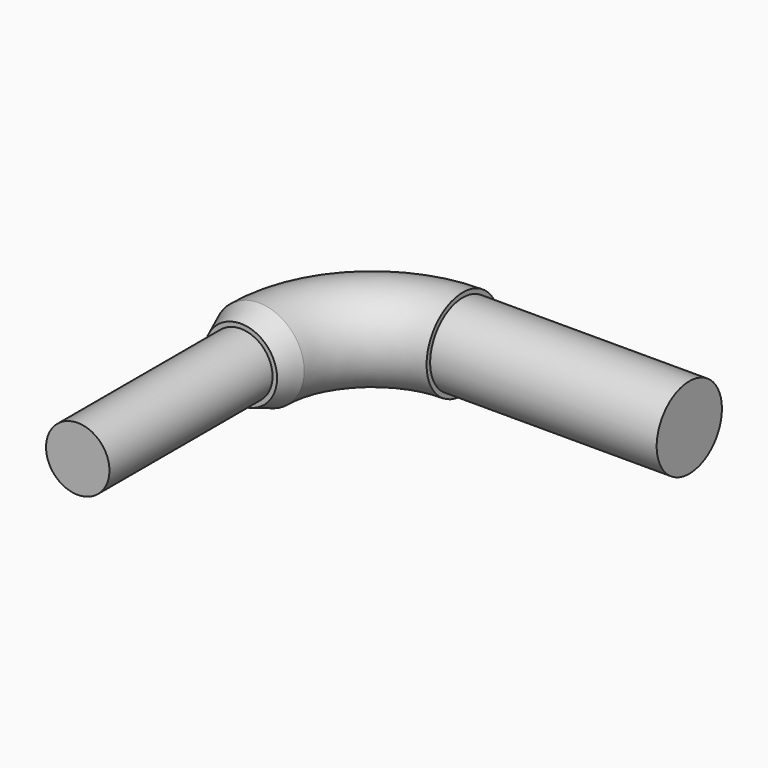
from build123d import *

# Parameters (mm, degrees)
F0_R     = 10
F3_ANGLE = 90
F4_R     = 7
F5_DEPTH = 50
F6_R     = 9
F7_DEPTH = 50
F8_DEPTH = 5
F9_SIZE2 = 4.99999
F9_SIZE  = 1.99999


# Not quite as in the source:
# - a fillet or chamfer is up to 0.001 mm smaller than in the source, because OpenCascade refuses the exact size


with BuildPart() as f3:
    # F0 (on Front) → F3 (revolve)
    with BuildSketch(Plane.XZ):
        with Locations((-40.3583608249, 0)):
            Circle(F0_R)
    revolve(axis=Axis((-15.3583608249, 0, 6.4160241745), (0, 0, -1)), revolution_arc=F3_ANGLE)

    # F6 (on face) → F7 (join)
    with BuildSketch(Plane.YZ.offset(-15.3583608249)):
        with Locations((25, 0)):
            Circle(F6_R)
    extrude(amount=F7_DEPTH)

    # F8 (add): a face of the model
    f8_faces = [f3.faces().sort_by_distance(p)[0] for p in [
        (-40.3583608249, 0, 0),
    ]]


with BuildPart() as f5:
    # F4 (on face) → F5 (new body)
    with BuildSketch(Plane.XZ):
        with Locations((-40.3583608249, 0)):
            Circle(F4_R)
    extrude(amount=F5_DEPTH)


with BuildPart() as f3_1:
    add(f3.part)

    add(f5.part)  # F8 merges F5
    extrude(f8_faces, amount=F8_DEPTH)

    # F9 (size 2 and 5 in the source; OpenCascade refuses exactly that, so slightly less here)
    f9_edges = [f3_1.edges().sort_by_distance(p)[0] for p in [
        (-50.358361, -5, 0),
    ]]
    f9_side = f3_1.faces().sort_by_distance((-50.075518, -5, 0))[0]
    chamfer(f9_edges, length=F9_SIZE, length2=F9_SIZE2, reference=f9_side)


solid = f3_1.part
